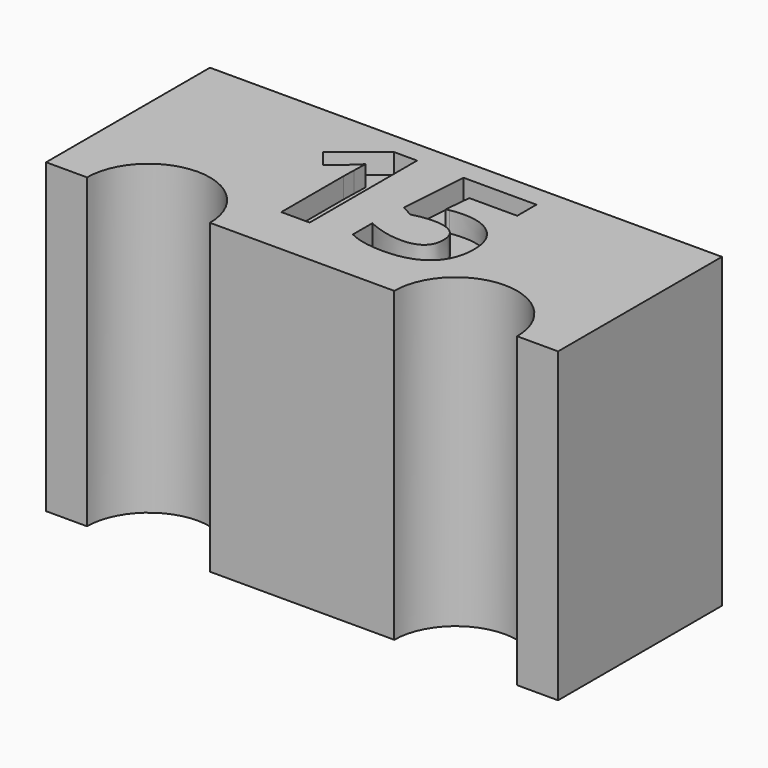
from build123d import *

# Parameters (mm, degrees)
F0_W         = 25
F0_H         = 10
F1_DEPTH     = 15
F2_R         = 3
F3_DEPTH     = 15.001
F4_TEXT_SIZE = 9.1828454232
F5_DEPTH     = 1


# Not quite as in the source:
# - Text() gives the source's letters only with a copy of the font that has no kerning and outlines rounded to 1/6400 em; it was checked with that copy


with BuildPart() as f1:
    # F0 (on Top) → F1 (new body)
    with BuildSketch(Plane.XY):
        Rectangle(F0_W, F0_H)
    extrude(amount=F1_DEPTH)

    # F2 (on Top) → F3 (cut, through all)
    with BuildSketch(Plane.XY):
        with Locations((-7.5, -5)):
            Circle(F2_R)
        with Locations((7.5, -5)):
            Circle(F2_R)
    extrude(amount=F3_DEPTH, mode=Mode.SUBTRACT)

    # F4 (on face) → F5 (cut)
    with BuildSketch(Plane.XY.offset(15)):
        with Locations((-5.3332244435, -2.6116487047)):
            Text('15', F4_TEXT_SIZE, font='Open Sans', font_style=FontStyle.BOLD, text_align=(TextAlign.LEFT, TextAlign.BOTTOM))
    extrude(amount=-F5_DEPTH, mode=Mode.SUBTRACT)


solid = f1.part
